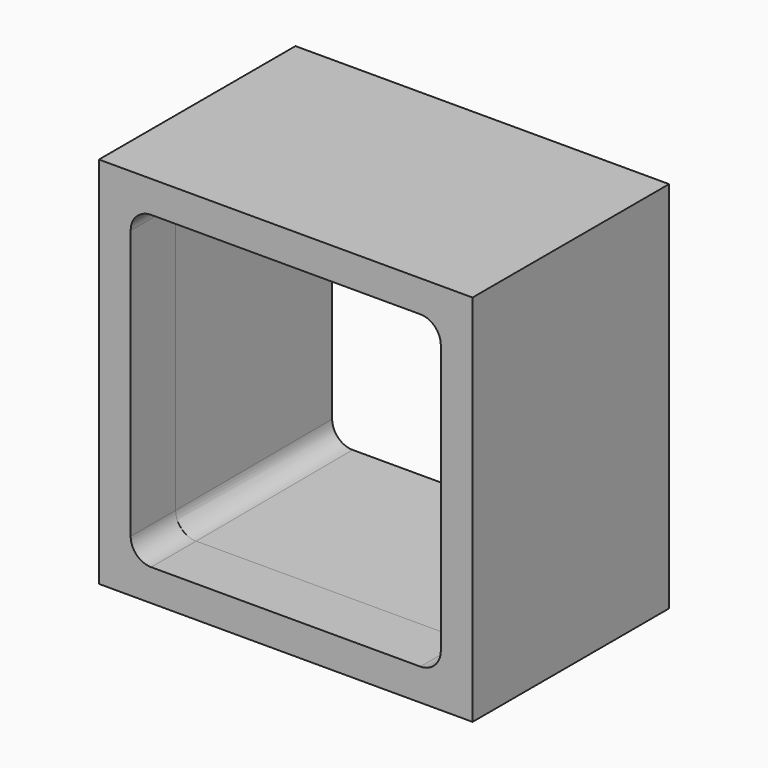
from build123d import *

# Parameters (mm, degrees)
F0_W     = 36.5
F0_H     = 36.5
F5_DEPTH = 24
F4_W     = 29.3
F4_H     = 29.3
F6_DEPTH = 19
F6_TAPER = -1.5074
F2_W     = 30.3
F2_H     = 30.3
F7_DEPTH = 5.501
F8_R     = 2
F8_R_2   = 1.999


# Not quite as in the source:
# - a fillet or chamfer is up to 0.001 mm smaller than in the source, because OpenCascade refuses the exact size


with BuildPart() as f5:
    # F0 (on Front) → F5 (new body)
    with BuildSketch(Plane.XZ):
        with Locations((-18.25, 18.25)):
            Rectangle(F0_W, F0_H)
    extrude(amount=-F5_DEPTH)

    # F4 (on offset) → F6 (cut)
    with BuildSketch(Plane.XZ.offset(-24.5)):
        with Locations((-18.25, 18.25)):
            Rectangle(F4_W, F4_H)
    extrude(amount=F6_DEPTH, taper=F6_TAPER, mode=Mode.SUBTRACT)

    # F2 (on offset) → F7 (cut, through all)
    with BuildSketch(Plane.XZ.offset(-5.5)):
        with Locations((-18.25, 18.25)):
            Rectangle(F2_W, F2_H)
    extrude(amount=F7_DEPTH, mode=Mode.SUBTRACT)

    # F8 (call 1 of 8: OpenCascade refuses the feature's edges together)
    f8_edges = [f5.edges().sort_by_distance(p)[0] for p in [
        (-3.343427, 14.75, 33.156573),
    ]]
    fillet(f8_edges, radius=F8_R)

    # F8#2 (call 2 of 8) (radius 2 in the source; OpenCascade refuses exactly that, so slightly less here)
    f8_2_edges = [f5.edges().sort_by_distance(p)[0] for p in [
        (-3.1, 2.75, 33.4),
    ]]
    fillet(f8_2_edges, radius=F8_R_2)

    # F8#3 (call 3 of 8)
    f8_3_edges = [f5.edges().sort_by_distance(p)[0] for p in [
        (-33.156573, 14.75, 3.343427),
    ]]
    fillet(f8_3_edges, radius=F8_R)

    # F8#4 (call 4 of 8) (radius 2 in the source; OpenCascade refuses exactly that, so slightly less here)
    f8_4_edges = [f5.edges().sort_by_distance(p)[0] for p in [
        (-33.4, 2.75, 3.1),
    ]]
    fillet(f8_4_edges, radius=F8_R_2)

    # F8#5 (call 5 of 8)
    f8_5_edges = [f5.edges().sort_by_distance(p)[0] for p in [
        (-33.156573, 14.75, 33.156573),
    ]]
    fillet(f8_5_edges, radius=F8_R)

    # F8#6 (call 6 of 8) (radius 2 in the source; OpenCascade refuses exactly that, so slightly less here)
    f8_6_edges = [f5.edges().sort_by_distance(p)[0] for p in [
        (-33.4, 2.75, 33.4),
    ]]
    fillet(f8_6_edges, radius=F8_R_2)

    # F8#7 (call 7 of 8)
    f8_7_edges = [f5.edges().sort_by_distance(p)[0] for p in [
        (-3.343427, 14.75, 3.343427),
    ]]
    fillet(f8_7_edges, radius=F8_R)

    # F8#8 (call 8 of 8) (radius 2 in the source; OpenCascade refuses exactly that, so slightly less here)
    f8_8_edges = [f5.edges().sort_by_distance(p)[0] for p in [
        (-3.1, 2.75, 3.1),
    ]]
    fillet(f8_8_edges, radius=F8_R_2)


solid = f5.part
